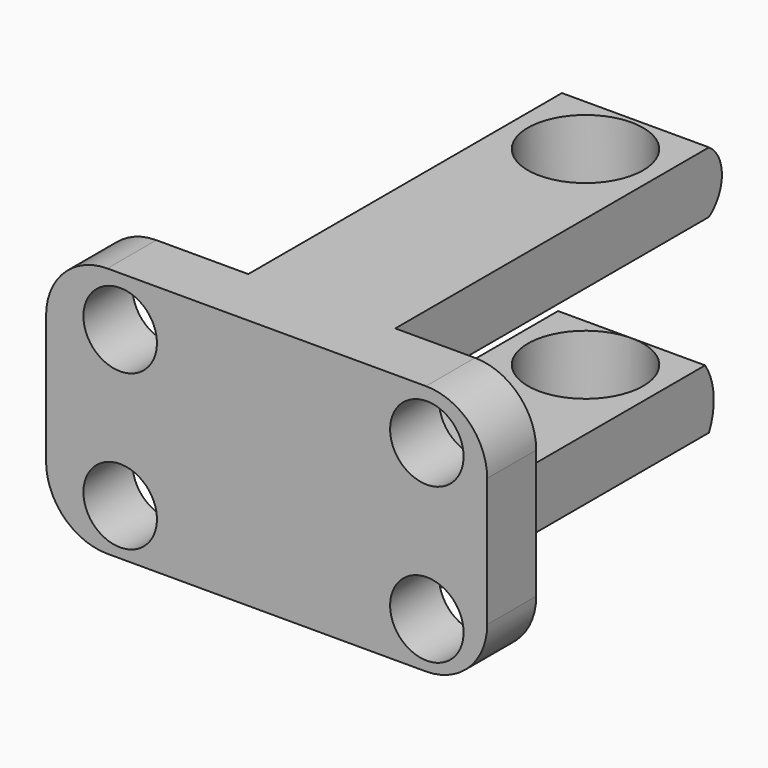
from build123d import *

# Parameters (mm, degrees)
F1_DEPTH = 5
F3_DEPTH = 6
F4_R     = 3
F5_DEPTH = 5
F6_R     = 4.7014922297
F7_DEPTH = 25


# Not quite as in the source:
# - a feature names something its author has since deleted; it is built from what else it names


with BuildPart() as f1:
    # F0 (on Front) → F1 (new body)
    with BuildSketch(Plane.XZ):
        with BuildLine():
            Line((-13.5, 0), (0, 0))
            Line((0, 0), (12.5000002478, 0))
            ThreePointArc((12.5000002478, 0), (16.0355341537, 1.4644660941), (17.5000002478, 5))
            Line((17.5000002478, 5), (17.5000002478, 15.5))
            ThreePointArc((17.5000002478, 15.5), (16.0355341537, 19.0355339059), (12.5000002478, 20.5))
            Line((12.5000002478, 20.5), (0, 20.5))
            Line((0, 20.5), (-13.5, 20.5))
            ThreePointArc((-13.5, 20.5), (-17.0355339059, 19.0355339059), (-18.5, 15.5))
            Line((-18.5, 15.5), (-18.5, 5))
            ThreePointArc((-18.5, 5), (-17.0355339059, 1.4644660941), (-13.5, 0))
        make_face()
    extrude(amount=F1_DEPTH)

    # F2 (on Right) → F3 (join, symmetric)
    with BuildSketch(Plane.YZ):
        with BuildLine():
            Line((0, 4.0980060585), (0, 0))
            Line((0, 0), (32, 0))
            ThreePointArc((32, 0), (32.4704336179, 2.5533766687), (31.6014834029, 5))
            Line((31.6014834029, 5), (22.881918614, 5))
            Line((22.881918614, 5), (0, 5))
            Line((0, 5), (0, 4.0980060585))
        make_face()
        with BuildLine():
            Line((32, 20.5), (0, 20.5))
            Line((0, 20.5), (0, 15.5))
            Line((0, 15.5), (32, 15.5))
            ThreePointArc((32, 15.5), (33.3190218942, 18), (32, 20.5))
        make_face()
    extrude(amount=F3_DEPTH, both=True)

    # F4 (on face) → F5 (cut)
    with BuildSketch(Plane(origin=(0, 0, 0), x_dir=(-1, 0, 0), z_dir=(0, 1, 0))):
        with Locations((12.4534495048, 16.4442711417)):
            Circle(F4_R)
        with Locations((12.4534495048, 3.7959093649)):
            Circle(F4_R)
        with Locations((-12.5748278123, 16.4442711417)):
            Circle(F4_R)
        with Locations((-12.5748278123, 3.7959093649)):
            Circle(F4_R)
    extrude(amount=-F5_DEPTH, mode=Mode.SUBTRACT)

    # F6 (on face) → F7 (cut)
    with BuildSketch(Plane.XY.offset(20.5)):
        with Locations((0, 26.9046556205)):
            Circle(F6_R)
    extrude(amount=-F7_DEPTH, mode=Mode.SUBTRACT)


solid = f1.part
